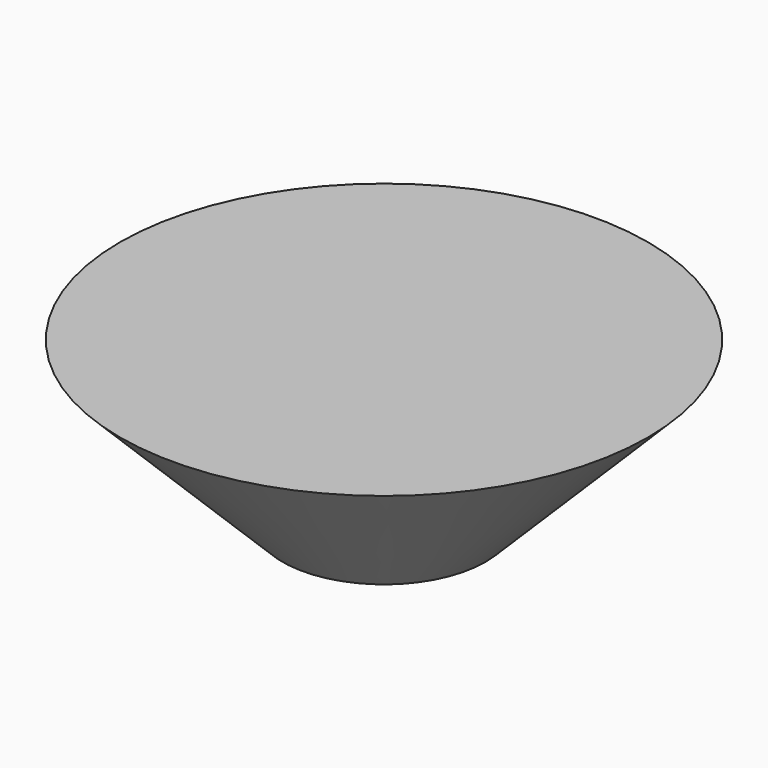
from build123d import *

# Parameters (mm, degrees)
F0_R     = 3.81
F1_DEPTH = 2.032


# Not quite as in the source:
# - a fillet or chamfer that OpenCascade refuses, or shapes differently, is made with other operations: its cross-section is extruded or revolved along the edge and cut away or added


with BuildPart() as f1:
    # F0 (on Top) → F1 (new body)
    with BuildSketch(Plane.XY):
        Circle(F0_R)
    extrude(amount=-F1_DEPTH)

    # F2: chamfer of 2.54 on 1 edges, made by hand

    # F2_s1 → F2_t2 (revolve, cut)
    with BuildSketch(Plane.XZ):
        Polygon((3.81, 0.508), (1.27, -2.032), (3.81, -2.032), align=None)
    revolve(axis=Axis((0, 0, -2.032), (0, 0, 1)), mode=Mode.SUBTRACT)


solid = f1.part
